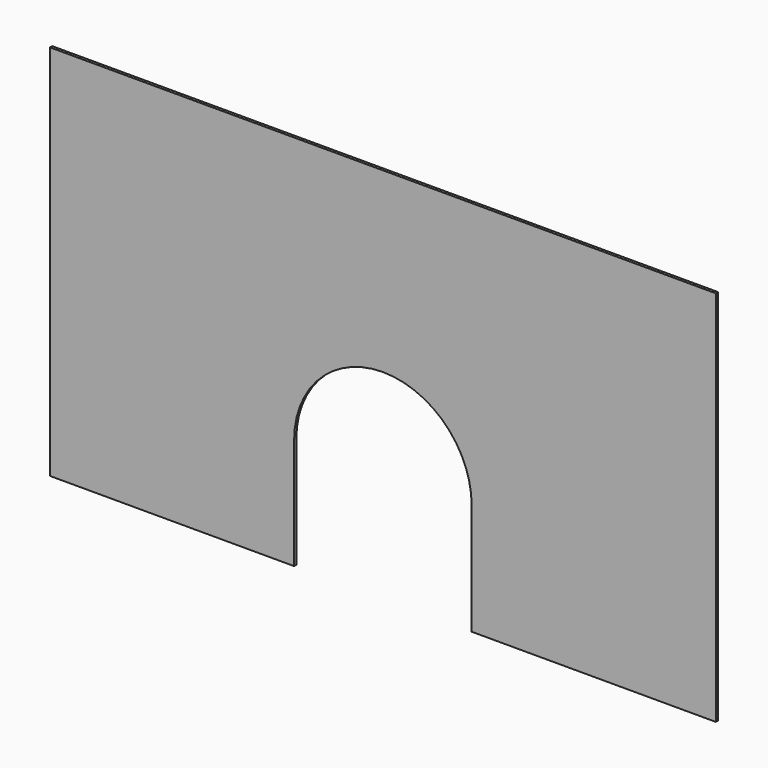
from build123d import *

# Parameters (mm, degrees)
F1_DEPTH = 3.175


# Not quite as in the source:
# - a length typed as a fraction of an inch, garbled in the dataset ("3 / 203.2 mm" for 3/8 in), is restored


with BuildPart() as f1:
    # F0 (on Front) → F1 (new body)
    with BuildSketch(Plane.XZ):
        with BuildLine():
            Line((381, -215.9), (381, 215.9))
            Line((381, 215.9), (-381, 215.9))
            Line((-381, 215.9), (-381, -215.9))
            Line((-381, -215.9), (-101.6, -215.9))
            Line((-101.6, -215.9), (-101.6, -88.9))
            ThreePointArc((-101.6, -88.9), (0, 12.7), (101.6, -88.9))
            Line((101.6, -88.9), (101.6, -215.9))
            Line((101.6, -215.9), (381, -215.9))
        make_face()
    extrude(amount=F1_DEPTH)


solid = f1.part
